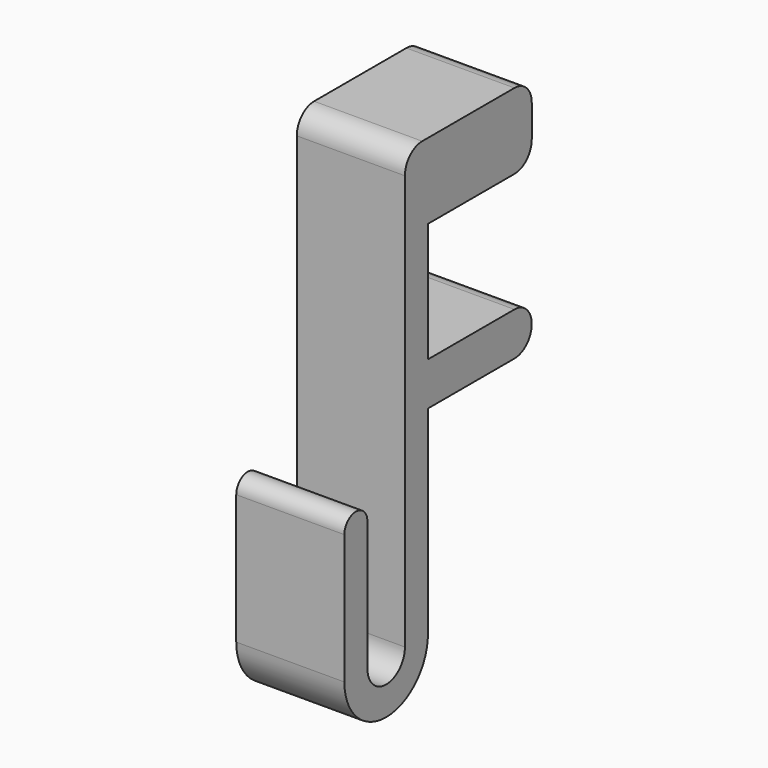
from build123d import *

# Parameters (mm, degrees)
F1_DEPTH = 15
F2_R     = 2.99999


# Not quite as in the source:
# - a fillet or chamfer is up to 0.001 mm smaller than in the source, because OpenCascade refuses the exact size


with BuildPart() as f1:
    # F0 (on Right) → F1 (new body)
    with BuildSketch(Plane.YZ):
        with BuildLine():
            Line((-18, 30.3650735612), (0, 30.3650735612))
            Line((0, 30.3650735612), (0, 40.8650735612))
            Line((0, 40.8650735612), (-22, 40.8650735612))
            Line((-22, 40.8650735612), (-22, -19.700880742))
            ThreePointArc((-22, -19.700880742), (-25.25, -22.950880742), (-28.5, -19.700880742))
            Line((-28.5, -19.700880742), (-28.5, -1.700880742))
            ThreePointArc((-28.5, -1.700880742), (-30.5, 0.299119258), (-32.5, -1.700880742))
            Line((-32.5, -1.700880742), (-32.5, -19.700880742))
            ThreePointArc((-32.5, -19.700880742), (-25.25, -26.950880742), (-18, -19.700880742))
            Line((-18, -19.700880742), (-18, 7.8150735612))
            Line((-18, 7.8150735612), (0, 7.8150735612))
            Line((0, 7.8150735612), (0, 13.8150735612))
            Line((0, 13.8150735612), (-18, 13.8150735612))
            Line((-18, 13.8150735612), (-18, 30.3650735612))
        make_face()
    extrude(amount=F1_DEPTH)

    # F2 (radius 3 in the source; OpenCascade refuses exactly that, so slightly less here)
    f2_edges = [f1.edges().sort_by_distance(p)[0] for p in [
        (7.5, 0, 30.365074),
        (7.5, 0, 13.815074),
        (7.5, 0, 40.865074),
        (7.5, 0, 7.815074),
        (7.5, -22, 40.865074),
    ]]
    fillet(f2_edges, radius=F2_R)


solid = f1.part
